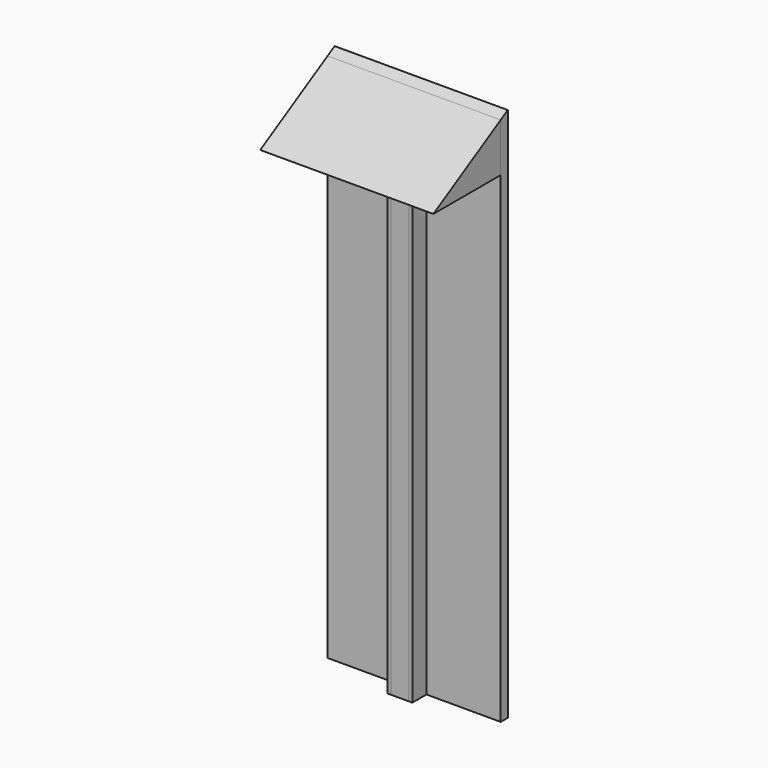
from build123d import *

# Parameters (mm, degrees)
F0_W          = 50
F0_H          = 1500
F1_DEPTH      = 50
F2_W          = 50
F2_H          = 1500
F3_DEPTH      = 10
F4_W          = 50
F4_H          = 1500
F5_DEPTH      = 10
F7_DEPTH      = 25
F9_DEPTH      = 100
F11_DEPTH     = 490
F12_W         = 8
F12_H         = 200
F12_TEXT_SIZE = 208.3333333333
F13_DEPTH     = 10
F15_DEPTH     = 490


# Not quite as in the source:
# - Text() gives the source's letters only with a copy of the font that has no kerning and outlines rounded to 1/6400 em; it was checked with that copy


with BuildPart() as f1:
    # F0 (on Front) → F1 (new body)
    with BuildSketch(Plane.XZ):
        Rectangle(F0_W, F0_H)
    extrude(amount=F1_DEPTH)


with BuildPart() as f3:
    # F2 (on face) → F3 (new body)
    with BuildSketch(Plane(origin=(-25, 0, 0), x_dir=(0, -1, 0), z_dir=(-1, 0, 0))):
        with Locations((25, 0)):
            Rectangle(F2_W, F2_H)
    extrude(amount=F3_DEPTH)


with BuildPart() as f5:
    # F4 (on face) → F5 (new body)
    with BuildSketch(Plane.YZ.offset(25)):
        with Locations((-25, 0)):
            Rectangle(F4_W, F4_H)
    extrude(amount=F5_DEPTH)


with BuildPart() as f7:
    # F6 (on face) → F7 (new body)
    with BuildSketch(Plane(origin=(0, 0, 0), x_dir=(-1, 0, 0), z_dir=(0, 1, 0))):
        Polygon((-245, 750), (-245, 500), (-245, -500), (-245, -750), (245, -750), (245, -500), (245, 500), (245, 750), align=None)
    extrude(amount=F7_DEPTH)

    # F10 (on face) → F11 (join)
    with BuildSketch(Plane.YZ.offset(245)):
        Polygon((25, 764.4337567297), (0, 750), (25, 750), align=None)
    extrude(amount=-F11_DEPTH)


with BuildPart() as f9_tool:
    # F8 (on face) → F9 (new body)
    with BuildSketch(Plane.YZ.offset(35)):
        Polygon((-50, 721.1324865405), (0, 750), (-50, 750), align=None)
    extrude(amount=-F9_DEPTH)


with BuildPart() as f1_1:
    add(f1.part)

    # F9: cut by f9_tool
    add(f9_tool.part, mode=Mode.SUBTRACT)


with BuildPart() as f3_1:
    add(f3.part)

    # F9: cut by f9_tool
    add(f9_tool.part, mode=Mode.SUBTRACT)


with BuildPart() as f5_1:
    add(f5.part)

    # F9: cut by f9_tool
    add(f9_tool.part, mode=Mode.SUBTRACT)


with BuildPart() as f13:
    # F12 (on face) → F13 (new body)
    with BuildSketch(Plane(origin=(0, 25, 0), x_dir=(-1, 0, 0), z_dir=(0, 1, 0))):
        with Locations((-69.8317065835, 215.8840387032)):
            Rectangle(F12_W, F12_H)
        with Locations((47.6211793721, 215.8840387032)):
            Rectangle(F12_W, F12_H)
        with Locations((-186.962890625, 140.8840387032)):
            Text('SEB', F12_TEXT_SIZE, font='Open Sans', font_style=FontStyle.BOLD, text_align=(TextAlign.LEFT, TextAlign.BOTTOM))
    extrude(amount=F13_DEPTH)


with BuildPart() as f15:
    # F14 (on face) → F15 (new body)
    with BuildSketch(Plane.YZ.offset(245)):
        Polygon((0, 612.5), (0, 750), (-238.1569860407, 612.5), align=None)
    extrude(amount=-F15_DEPTH)


solid = Compound([f7.part, f1_1.part, f3_1.part, f5_1.part, f13.part, f15.part])
